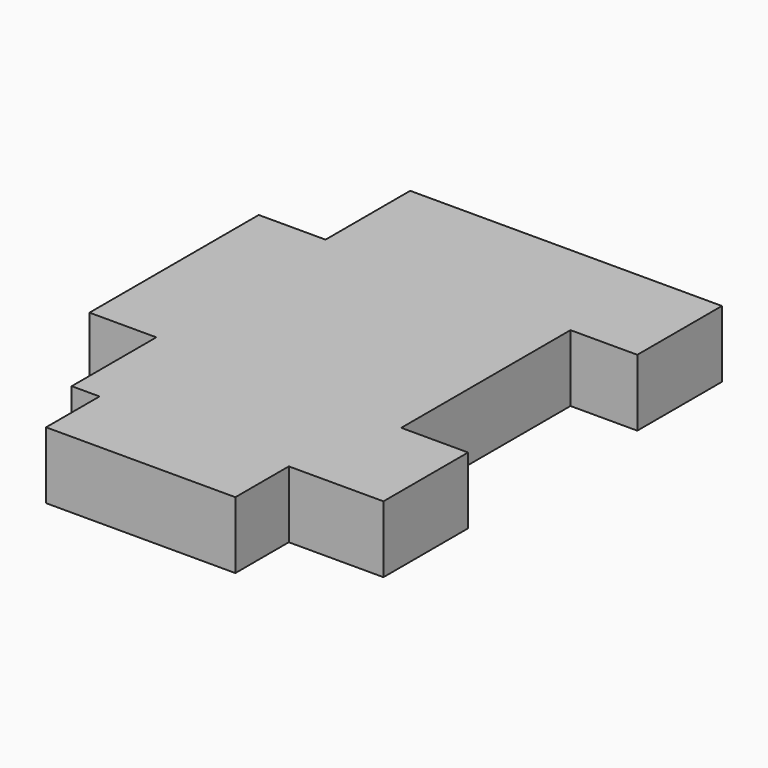
from build123d import *

# Parameters (mm, degrees)
F0_W     = 53.975
F0_H     = 19.05
F1_DEPTH = 19.05
F2_W     = 60.325
F2_H     = 19.05
F3_DEPTH = 19.05
F4_W     = 30.1625
F4_H     = 19.05
F5_DEPTH = 19.05


# Not quite as in the source:
# - a length typed as a fraction of an inch, garbled in the dataset ("3 / 203.2 mm" for 3/8 in), is restored


with BuildPart() as f1:
    # F0 (on Top) → F1 (new body)
    with BuildSketch(Plane.XY):
        Polygon((53.975, -60.325), (53.975, 60.325), (-53.975, 60.325), (-53.975, -60.325), (-26.9875, -60.325), (-26.9875, -41.275), (26.9875, -41.275), (26.9875, -60.325), align=None)
        with Locations((0, -69.85)):
            Rectangle(F0_W, F0_H)
        with Locations((0, -50.8)):
            Rectangle(F0_W, F0_H)
    extrude(amount=F1_DEPTH)

    # F2 (on face) → F3 (cut)
    with BuildSketch(Plane.YZ.offset(53.975)):
        with Locations((0, 9.525)):
            Rectangle(F2_W, F2_H)
    extrude(amount=-F3_DEPTH, mode=Mode.SUBTRACT)

    # F4 (on face) → F5 (cut)
    with BuildSketch(Plane(origin=(-53.975, 0, 0), x_dir=(0, -1, 0), z_dir=(-1, 0, 0))):
        with Locations((-45.24375, 9.525)):
            Rectangle(F4_W, F4_H)
        with Locations((45.24375, 9.525)):
            Rectangle(F4_W, F4_H)
    extrude(amount=-F5_DEPTH, mode=Mode.SUBTRACT)


solid = f1.part
